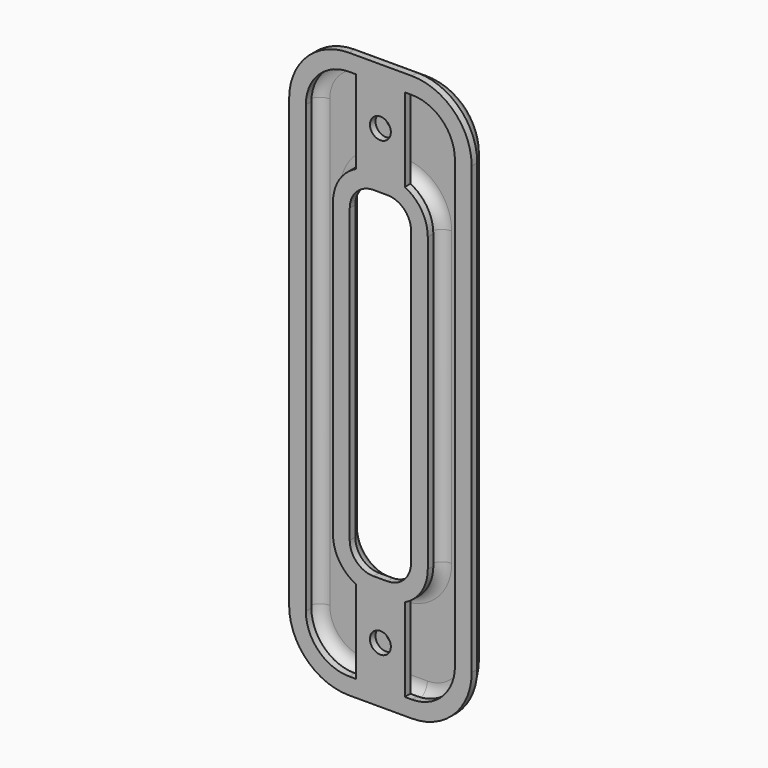
from build123d import *

# Parameters (mm, degrees)
F0_W     = 31.75
F0_H     = 101.6
F0_W_2   = 12.7
F0_H_2   = 63.5
F1_DEPTH = 3.81
F2_R     = 10.16
F3_R     = 5.08
F4_R     = 3.80999
F5_T     = 1.524
F6_R     = 1.905
F7_DEPTH = 1.524
F8_R     = 1.905
F9_DEPTH = 1.27


# Not quite as in the source:
# - a fillet or chamfer is up to 0.001 mm smaller than in the source, because OpenCascade refuses the exact size
# - a shell that OpenCascade refuses in one call is made with other operations: the cavity is built on its own and cut out


with BuildPart() as f1:
    # F0 (on Front) → F1 (new body)
    with BuildSketch(Plane.XZ):
        Rectangle(F0_W, F0_H)
        Rectangle(F0_W_2, F0_H_2, mode=Mode.SUBTRACT)
    extrude(amount=F1_DEPTH)

    # F2
    f2_edges = [f1.edges().sort_by_distance(p)[0] for p in [
        (-15.875, -1.905, 50.8),
        (15.875, -1.905, 50.8),
        (15.875, -1.905, -50.8),
        (-15.875, -1.905, -50.8),
    ]]
    fillet(f2_edges, radius=F2_R)

    # F3
    f3_edges = [f1.edges().sort_by_distance(p)[0] for p in [
        (-6.35, -1.905, 31.75),
        (6.35, -1.905, 31.75),
        (-6.35, -1.905, -31.75),
        (6.35, -1.905, -31.75),
    ]]
    fillet(f3_edges, radius=F3_R)

    # F4 (radius 3.81 in the source; OpenCascade refuses exactly that, so slightly less here)
    f4_edges = [f1.edges().sort_by_distance(p)[0] for p in [
        (15.875, 0, 0),
        (4.862102, 0, 30.262102),
    ]]
    fillet(f4_edges, radius=F4_R)

    # F5: shell of thickness 1.524, made by hand


with BuildPart() as f5_core1:
    # F5_t2: copy of F1
    add(f1.part)

    # the walls: a layer under each face that stays
    f5_faces = [f5_core1.faces().sort_by_distance(p)[0] for p in [
        (-10.3414371429, 0, -40.2771514286),
        (14.7590797653, -1.1159202347, 0),
        (12.1101301316, -1.1159202347, -47.0351301316),
        (12.1101301316, -1.1159202347, 47.0351301316),
        (0, -1.1159202347, -49.6840797653),
        (0, -1.1159202347, 49.6840797653),
        (-12.1101301316, -1.1159202347, -47.0351301316),
        (-12.1101301316, -1.1159202347, 47.0351301316),
        (-14.7590797653, -1.1159202347, 0),
        (5.6511772137, -1.1159202347, 31.0511772137),
        (0, -1.1159202347, 32.8659202347),
        (7.4659202347, -1.1159202347, 0),
        (-5.6511772137, -1.1159202347, 31.0511772137),
        (5.6511772137, -1.1159202347, -31.0511772137),
        (-7.4659202347, -1.1159202347, 0),
        (0, -1.1159202347, -32.8659202347),
        (-5.6511772137, -1.1159202347, -31.0511772137),
        (15.875, -3.809995, 0),
        (12.8992048969, -3.809995, -47.8242048969),
        (12.8992048969, -3.809995, 47.8242048969),
        (0, -3.809995, -50.8),
        (0, -3.809995, 50.8),
        (-12.8992048969, -3.809995, -47.8242048969),
        (-12.8992048969, -3.809995, 47.8242048969),
        (-15.875, -3.809995, 0),
        (4.8621024484, -3.809995, 30.2621024484),
        (0, -3.809995, 31.75),
        (6.35, -3.809995, 0),
        (-4.8621024484, -3.809995, 30.2621024484),
        (4.8621024484, -3.809995, -30.2621024484),
        (-6.35, -3.809995, 0),
        (0, -3.809995, -31.75),
        (-4.8621024484, -3.809995, -30.2621024484),
    ]]
    thicken(f5_faces, amount=-F5_T, mode=Mode.SUBTRACT)


with BuildPart() as f1_1:
    add(f1.part)

    # what is left inside the walls is the cavity
    f5_cavity = [f5_core1.part.solids().sort_by_distance(p)[0] for p in [
        (-7.9375, -3.79476, 16.933333),
    ]]
    add(f5_cavity, mode=Mode.SUBTRACT)

    # F6 (on face) → F7 (cut, through all)
    with BuildSketch(Plane(origin=(0, 0, 0), x_dir=(-1, 0, 0), z_dir=(0, 1, 0))):
        with Locations((0, 41.275)):
            Circle(F6_R)
        with Locations((0, -41.275)):
            Circle(F6_R)
    extrude(amount=-F7_DEPTH, mode=Mode.SUBTRACT)


with BuildPart() as f9:
    # F8 (on face) → F9 (new body)
    with BuildSketch(Plane.XZ.offset(3.81)):
        with BuildLine():
            ThreePointArc((-5.715, 51.5620000048), (-13.4380202658, 48.3630202672), (-16.637, 40.64))
            Line((-16.637, 40.64), (-16.637, -40.64))
            ThreePointArc((-16.637, -40.64), (-13.4380202641, -48.3630202641), (-5.715, -51.562))
            Line((-5.715, -51.562), (5.715, -51.562))
            ThreePointArc((5.715, -51.562), (13.4380202641, -48.3630202641), (16.637, -40.64))
            Line((16.637, -40.64), (16.637, 40.64))
            ThreePointArc((16.637, 40.64), (13.4380202658, 48.3630202672), (5.715, 51.5620000048))
            Line((5.715, 51.5620000048), (-5.715, 51.5620000048))
        make_face()
        with BuildLine():
            Line((-5.715, 48.514), (-4.445, 48.514))
            Line((-4.445, 48.514), (-4.445, 33.3166029669))
            ThreePointArc((-4.445, 33.3166029669), (-7.5007706586, 30.5987979078), (-8.636, 26.67))
            Line((-8.636, 26.67), (-8.636, -26.67))
            ThreePointArc((-8.636, -26.67), (-7.5007706586, -30.5987979078), (-4.445, -33.3166029669))
            Line((-4.445, -33.3166029669), (-4.445, -48.514))
            Line((-4.445, -48.514), (-5.715, -48.514))
            ThreePointArc((-5.715, -48.514), (-11.2827587951, -46.2077587951), (-13.589, -40.64))
            Line((-13.589, -40.64), (-13.589, 40.64))
            ThreePointArc((-13.589, 40.64), (-11.2827587951, 46.2077587951), (-5.715, 48.514))
        make_face(mode=Mode.SUBTRACT)
        with Locations((0, -41.275)):
            Circle(F8_R, mode=Mode.SUBTRACT)
        with BuildLine():
            Line((-5.588, -26.67), (-5.588, 26.67))
            ThreePointArc((-5.588, 26.67), (-4.3232870812, 29.7232870812), (-1.27, 30.988))
            Line((-1.27, 30.988), (1.27, 30.988))
            ThreePointArc((1.27, 30.988), (4.3232870812, 29.7232870812), (5.588, 26.67))
            Line((5.588, 26.67), (5.588, -26.67))
            ThreePointArc((5.588, -26.67), (4.3232870812, -29.7232870812), (1.27, -30.988))
            Line((1.27, -30.988), (-1.27, -30.988))
            ThreePointArc((-1.27, -30.988), (-4.3232870812, -29.7232870812), (-5.588, -26.67))
        make_face(mode=Mode.SUBTRACT)
        with BuildLine():
            Line((4.445, 33.3166029669), (4.445, 48.514))
            Line((4.445, 48.514), (5.715, 48.514))
            ThreePointArc((5.715, 48.514), (11.2827587951, 46.2077587951), (13.589, 40.64))
            Line((13.589, 40.64), (13.589, -40.64))
            ThreePointArc((13.589, -40.64), (11.2827587951, -46.2077587951), (5.715, -48.514))
            Line((5.715, -48.514), (4.445, -48.514))
            Line((4.445, -48.514), (4.445, -33.3166029669))
            ThreePointArc((4.445, -33.3166029669), (7.5007706586, -30.5987979078), (8.636, -26.67))
            Line((8.636, -26.67), (8.636, 26.67))
            ThreePointArc((8.636, 26.67), (7.5007706586, 30.5987979078), (4.445, 33.3166029669))
        make_face(mode=Mode.SUBTRACT)
        with Locations((0, 41.275)):
            Circle(F8_R, mode=Mode.SUBTRACT)
    extrude(amount=F9_DEPTH)


solid = Compound([f1_1.part, f9.part])
